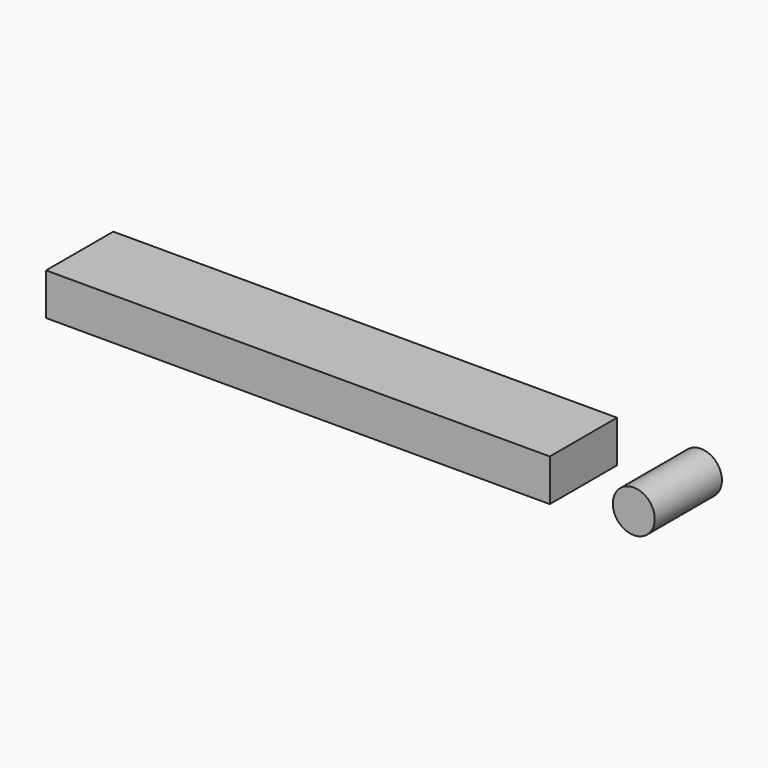
from build123d import *

# Parameters (mm, degrees)
F1_DEPTH = 50
F0_R     = 25


# Not quite as in the source:
# - a feature of the source that left no trace in its solid (it failed there, or was rolled back) is left out


with BuildPart() as f1:
    # F0 (on Front) → F1 (new body, symmetric)
    with BuildSketch(Plane.XZ):
        Polygon((-225, 25), (-300, 25), (-300, -25), (300, -25), (300, 25), (-195, 25), align=None)
    extrude(amount=F1_DEPTH, both=True)


with BuildPart() as f1b:
    # F0 (on Front) → F1, piece 2 (new body, symmetric)
    with BuildSketch(Plane.XZ):
        with Locations((400, 0)):
            Circle(F0_R)
    extrude(amount=F1_DEPTH, both=True)


solid = Compound([f1.part, f1b.part])
